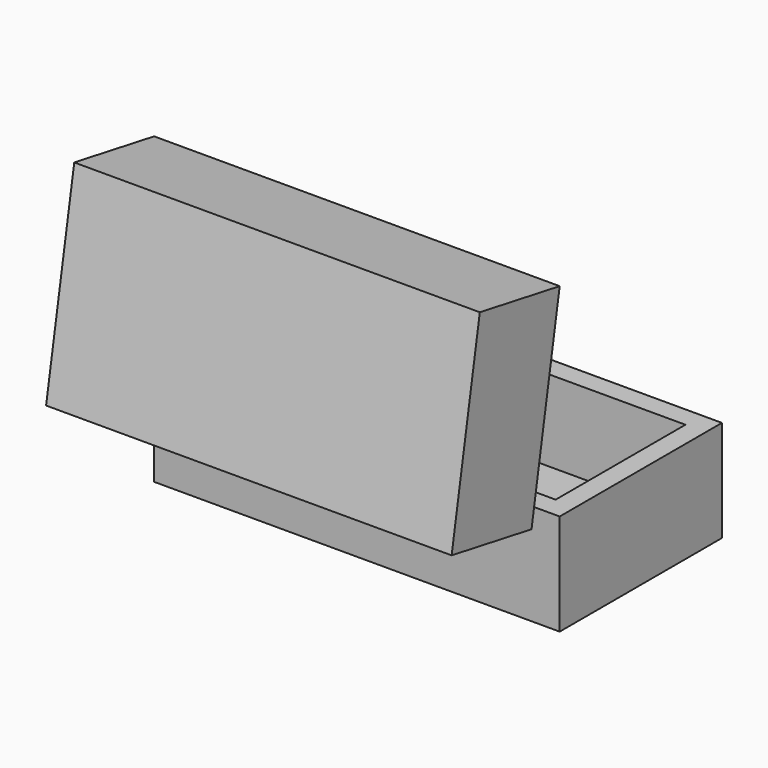
from build123d import *

# Parameters (mm, degrees)
F0_W     = 200
F0_H     = 100
F1_DEPTH = 50
F2_T     = -10
F4_ANGLE = 100


with BuildPart() as f1:
    # F0 (on Top) → F1 (new body)
    with BuildSketch(Plane.XY):
        Rectangle(F0_W, F0_H)
    extrude(amount=F1_DEPTH)

    # F2
    f2_openings = [f1.faces().sort_by_distance(p)[0] for p in [
        (0, 0, 50),
    ]]
    offset(amount=F2_T, openings=f2_openings)


with BuildPart() as f3_1:
    # F3: copy of F1
    add(f1.part.moved(Location((0, 0, 100))))


with BuildPart() as f3_1_1:
    # F4: moved
    add(f3_1.part.rotate(Axis((0, -50, 150), (-1, 0, 0)), F4_ANGLE))


solid = Compound([f1.part, f3_1_1.part])
